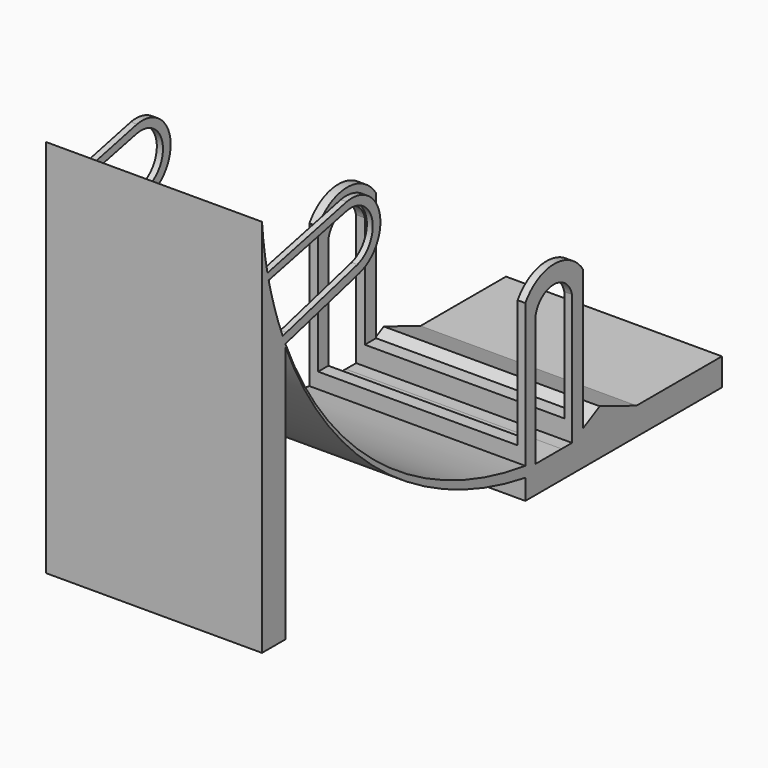
from build123d import *

# Parameters (mm, degrees)
F1_DEPTH = 25.4
F2_W     = 23.985484906
F2_H     = 10.9293945134
F3_DEPTH = 63.5
F4_DEPTH = 67.31
F5_W     = 23.835350119
F5_H     = 2.447379753
F6_DEPTH = 66.04
F7_W     = 23.4697095584
F7_H     = 17.8560893983
F8_DEPTH = 34.29


# Not quite as in the source:
# - the program builds the solid bodies; features that only make, move or delete a surface that nothing else refers to are left out


with BuildPart() as f1:
    # F0 (on Right) → F1 (new body)
    with BuildSketch(Plane.YZ):
        Polygon((0, 0), (0, 3.2231518999), (-12.5630013645, 3.2231518999), (-20.3921347857, 3.2231518999), (-20.3921347857, 0), align=None)
        Polygon((-20.3921347857, 3.2231518999), (-12.5630013645, 3.2231518999), (-17.9742891341, 5.361024756), (-20.3921347857, 4.0822205165), align=None)
        with BuildLine():
            Line((-20.3921347857, 0), (-20.3921347857, 3.2231518999))
            Line((-20.3921347857, 3.2231518999), (-22.0163828564, 3.2231518999))
            ThreePointArc((-22.0163828564, 3.2231518999), (-22.7959834692, 3.2163945029), (-23.575584082, 3.2231518999))
            Line((-23.575584082, 3.2231518999), (-27.4015981704, 3.2231518999))
            Line((-27.4015981704, 3.2231518999), (-28.9092455059, 3.2231518999))
            Line((-28.9092455059, 3.2231518999), (-28.9092455059, 2.3980058104))
            Line((-28.9092455059, 2.3980058104), (-28.9092455059, 0))
            Line((-28.9092455059, 0), (-20.3921347857, 0))
        make_face()
        Polygon((-22.0163828564, 3.2231518999), (-20.3921347857, 3.2231518999), (-20.3921347857, 4.0822205165), align=None)
        with BuildLine():
            Line((-22.0454800874, 3.2231518999), (-22.0163828564, 3.2231518999))
            Line((-22.0163828564, 3.2231518999), (-20.3921347857, 4.0822205165))
            Line((-20.3921347857, 4.0822205165), (-20.3921347857, 20.491162315))
            ThreePointArc((-20.3921347857, 20.491162315), (-24.6506901458, 22.8198511271), (-28.9092455059, 20.491162315))
            Line((-28.9092455059, 20.491162315), (-28.9092455059, 3.6338099802))
            ThreePointArc((-28.9092455059, 3.6338099802), (-28.1561856735, 3.5369589297), (-27.4015981704, 3.4528343954))
            Line((-27.4015981704, 3.4528343954), (-27.4015981704, 18.5859873891))
            ThreePointArc((-27.4015981704, 18.5859873891), (-24.7235391289, 20.7198764309), (-22.0454800874, 18.5859873891))
            Line((-22.0454800874, 18.5859873891), (-22.0454800874, 3.2231518999))
        make_face()
        with BuildLine():
            ThreePointArc((-64.1917986715, 30.3313969183), (-50.16224019, 11.8027548597), (-28.9092455059, 2.3980058104))
            Line((-28.9092455059, 2.3980058104), (-28.9092455059, 3.2231518999))
            Line((-28.9092455059, 3.2231518999), (-28.9092455059, 3.6338099802))
            ThreePointArc((-28.9092455059, 3.6338099802), (-50.1126919116, 12.4626789581), (-64.1917986715, 30.6096847649))
            Line((-64.1917986715, 30.6096847649), (-64.1917986715, 30.3313969183))
        make_face()
        with BuildLine():
            Line((-28.9092455059, 3.2231518999), (-27.4015981704, 3.2231518999))
            Line((-27.4015981704, 3.2231518999), (-27.4015981704, 3.4528343954))
            ThreePointArc((-27.4015981704, 3.4528343954), (-28.1561856735, 3.5369589297), (-28.9092455059, 3.6338099802))
            Line((-28.9092455059, 3.6338099802), (-28.9092455059, 3.2231518999))
        make_face()
        with BuildLine():
            ThreePointArc((-67.6309564566, 44.6495479383), (-66.4828080231, 37.35321731), (-64.1917986715, 30.3313969183))
            Line((-64.1917986715, 30.3313969183), (-64.1917986715, 30.6096847649))
            ThreePointArc((-64.1917986715, 30.6096847649), (-64.3937854186, 31.0930746092), (-64.59012772, 31.5787844899))
            ThreePointArc((-64.59012772, 31.5787844899), (-65.5320044676, 34.1785482504), (-66.3123383407, 36.8312793835))
            ThreePointArc((-66.3123383407, 36.8312793835), (-66.4844767509, 37.5124245346), (-66.645954144, 38.1961755131))
            ThreePointArc((-66.645954144, 38.1961755131), (-66.7377613235, 38.6078575578), (-66.8257035474, 39.0203825019))
            ThreePointArc((-66.8257035474, 39.0203825019), (-67.3173861233, 41.8222257294), (-67.6309564566, 44.6495479383))
        make_face()
        with BuildLine():
            Line((-64.1917986715, 0), (-64.1917986715, 30.3313969183))
            ThreePointArc((-64.1917986715, 30.3313969183), (-66.4828080231, 37.35321731), (-67.6309564566, 44.6495479383))
            Line((-67.6309564566, 44.6495479383), (-67.6309564566, 0))
            Line((-67.6309564566, 0), (-64.1917986715, 0))
        make_face()
        with BuildLine():
            ThreePointArc((-64.59012772, 31.5787844899), (-64.3937854186, 31.0930746092), (-64.1917986715, 30.6096847649))
            Line((-64.1917986715, 30.6096847649), (-64.0304028831, 31.7278995465))
            Line((-64.0304028831, 31.7278995465), (-64.59012772, 31.5787844899))
        make_face()
        with BuildLine():
            Line((-64.0304028831, 31.7278995465), (-64.1917986715, 30.6096847649))
            Line((-64.1917986715, 30.6096847649), (-53.3271447245, 33.5041132079))
            ThreePointArc((-53.3271447245, 33.5041132079), (-50.3228913796, 38.4738529349), (-55.1768802106, 41.6617430747))
            Line((-55.1768802106, 41.6617430747), (-66.8257035474, 39.0203825019))
            ThreePointArc((-66.8257035474, 39.0203825019), (-66.7377613235, 38.6078575578), (-66.645954144, 38.1961755131))
            Line((-66.645954144, 38.1961755131), (-55.2403122474, 40.7000877275))
            ThreePointArc((-55.2403122474, 40.7000877275), (-51.4541715224, 38.3935253272), (-53.5909704186, 34.5090456743))
            Line((-53.5909704186, 34.5090456743), (-64.0304028831, 31.7278995465))
        make_face()
    extrude(amount=F1_DEPTH)

    # F2 (on Front) → F3 (cut)
    with BuildSketch(Plane.XZ):
        with Locations((12.7173874935, 37.006566301)):
            Rectangle(F2_W, F2_H)
    extrude(amount=F3_DEPTH, mode=Mode.SUBTRACT)

    # F2 (on Front) → F4 (cut)
    with BuildSketch(Plane.XZ):
        with Locations((12.7173874935, 37.006566301)):
            Rectangle(F2_W, F2_H)
    extrude(amount=F4_DEPTH, mode=Mode.SUBTRACT)

    # F5 (on Front) → F6 (cut)
    with BuildSketch(Plane.XZ):
        with Locations((12.7131266927, 31.5032089129)):
            Rectangle(F5_W, F5_H)
    extrude(amount=F6_DEPTH, mode=Mode.SUBTRACT)

    # F7 (on Front) → F8 (cut)
    with BuildSketch(Plane.XZ):
        with Locations((12.7604022855, 14.3902720883)):
            Rectangle(F7_W, F7_H)
    extrude(amount=F8_DEPTH, mode=Mode.SUBTRACT)


solid = f1.part
